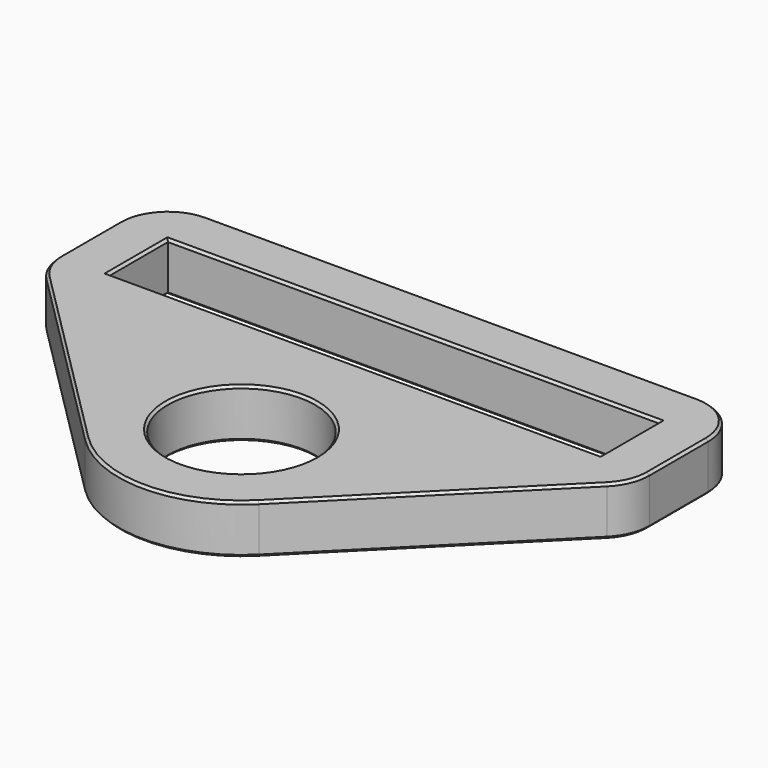
from build123d import *

# Parameters (mm, degrees)
F0_W        = 2
F0_H        = 2
F0_W_2      = 20
F0_H_2      = 3
F1_DEPTH    = 2
F2_T1_DEPTH = 12
F2_T3_DEPTH = 6.1421356237
F3_SIZE     = 0.1


# Not quite as in the source:
# - a fillet or chamfer that OpenCascade refuses, or shapes differently, is made with other operations: its cross-section is extruded or revolved along the edge and cut away or added


with BuildPart() as f1:
    # F0 (on Top) → F1 (new body)
    with BuildSketch(Plane.XY):
        with Locations((-11, 2.5)):
            Rectangle(F0_W, F0_H)
        with Locations((0, 2.5)):
            Rectangle(F0_W_2, F0_H)
        with Locations((11, 2.5)):
            Rectangle(F0_W, F0_H)
        with Locations((11, 0)):
            Rectangle(F0_W, F0_H_2)
        Polygon((12, -1.5), (10, -1.5), (11.4142135624, -2.9142135624), (12, -2.3284271247), align=None)
        Polygon((11.4142135624, -2.9142135624), (10, -1.5), (2.1213203436, -9.3786796564), (3.5355339059, -10.7928932188), align=None)
        with BuildLine():
            ThreePointArc((2.1213203436, -9.3786796564), (0, -10.2573593129), (-2.1213203436, -9.3786796564))
            Line((-2.1213203436, -9.3786796564), (-3.5355339059, -10.7928932188))
            ThreePointArc((-3.5355339059, -10.7928932188), (0, -12.2573593129), (3.5355339059, -10.7928932188))
            Line((3.5355339059, -10.7928932188), (2.1213203436, -9.3786796564))
        make_face()
        Polygon((-2.1213203436, -9.3786796564), (-10, -1.5), (-11.4142135624, -2.9142135624), (-3.5355339059, -10.7928932188), align=None)
        Polygon((-11.4142135624, -2.9142135624), (-10, -1.5), (-12, -1.5), (-12, -2.3284271247), align=None)
        with Locations((-11, 0)):
            Rectangle(F0_W, F0_H_2)
        with BuildLine():
            Line((0, -1.5), (-10, -1.5))
            Line((-10, -1.5), (-2.1213203436, -9.3786796564))
            ThreePointArc((-2.1213203436, -9.3786796564), (-1.1480502971, -4.4857207153), (3, -7.2573593129))
            ThreePointArc((3, -7.2573593129), (2.7716385975, -8.40540961), (2.1213203436, -9.3786796564))
            Line((2.1213203436, -9.3786796564), (10, -1.5))
            Line((10, -1.5), (0, -1.5))
        make_face()
    extrude(amount=F1_DEPTH)

    # F2: fillet of radius 2 on 4 edges, made by hand

    # F2_s2 → F2_t1 (cut)
    with BuildSketch(Plane.XY.offset(-5)):
        with BuildLine():
            ThreePointArc((-10, 3.5), (-11.4142135624, 2.9142135624), (-12, 1.5))
            Line((-12, 1.5), (-12, 3.5))
            Line((-12, 3.5), (-10, 3.5))
        make_face()
        with BuildLine():
            ThreePointArc((12, 1.5), (11.4142135624, 2.9142135624), (10, 3.5))
            Line((10, 3.5), (12, 3.5))
            Line((12, 3.5), (12, 1.5))
        make_face()
    extrude(amount=F2_T1_DEPTH, mode=Mode.SUBTRACT)

    # F2_s4 → F2_t3 (cut)
    with BuildSketch(Plane.XY.offset(-2.0710678119)):
        with BuildLine():
            ThreePointArc((-11.4142135624, -2.9142135624), (-11.847759065, -2.2653668647), (-12, -1.5))
            Line((-12, -1.5), (-12, -2.3284271247))
            Line((-12, -2.3284271247), (-11.4142135624, -2.9142135624))
        make_face()
        with BuildLine():
            ThreePointArc((11.4142135624, -2.9142135624), (11.847759065, -2.2653668647), (12, -1.5))
            Line((12, -1.5), (12, -2.3284271247))
            Line((12, -2.3284271247), (11.4142135624, -2.9142135624))
        make_face()
    extrude(amount=F2_T3_DEPTH, mode=Mode.SUBTRACT)

    # F3
    f3_edges = [f1.edges().sort_by_distance(p)[0] for p in [
        (-11.414214, 2.914214, 2),
        (0, 3.5, 2),
        (11.414214, 2.914214, 2),
        (12, 0, 2),
        (11.847759, -2.265367, 2),
        (7.474874, -6.853553, 2),
        (0, -12.257359, 2),
        (-7.474874, -6.853553, 2),
        (-11.847759, -2.265367, 2),
        (-12, 0, 2),
        (2.12132, -5.136039, 2),
        (0, 1.5, 2),
        (-10, 0, 2),
        (10, 0, 2),
        (0, -1.5, 2),
        (-11.414214, 2.914214, 0),
        (0, 3.5, 0),
        (11.414214, 2.914214, 0),
        (12, 0, 0),
        (11.847759, -2.265367, 0),
        (7.474874, -6.853553, 0),
        (0, -12.257359, 0),
        (-7.474874, -6.853553, 0),
        (-11.847759, -2.265367, 0),
        (-12, 0, 0),
        (2.12132, -5.136039, 0),
        (0, 1.5, 0),
        (-10, 0, 0),
        (10, 0, 0),
        (0, -1.5, 0),
    ]]
    chamfer(f3_edges, length=F3_SIZE)


solid = f1.part
